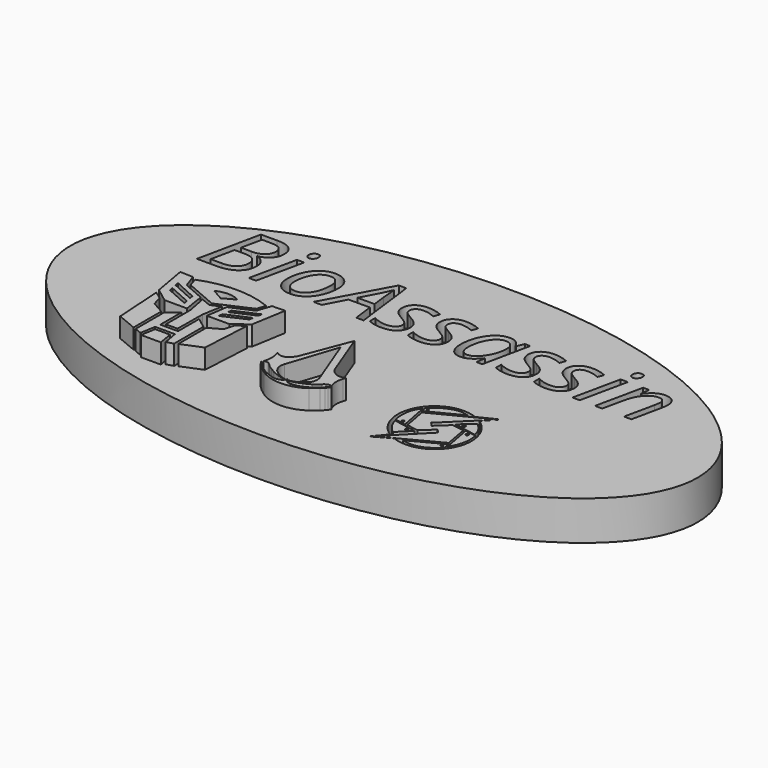
from build123d import *

# Parameters (mm, degrees)
F1_DEPTH     = 6.35
F3_DEPTH     = 3.175
F4_TEXT_SIZE = 14.3641968154
F5_DEPTH     = 3.175
F7_DEPTH     = 3.175
F8_R         = 0.1916506527
F8_R_2       = 0.1928443089
F8_R_3       = 0.2170281885
F8_R_4       = 0.2291424011
F8_R_5       = 0.2516270003
F8_R_6       = 0.1916500299
F9_DEPTH     = 3.175


# Not quite as in the source:
# - Text() gives the source's letters only with a copy of the font that has no kerning and outlines rounded to 1/6400 em; it was checked with that copy


with BuildPart() as f1:
    # F0 (on Top) → F1 (new body)
    with BuildSketch(Plane.XY):
        with BuildLine():
            add(Edge.make_bspline(
                [(-2.0761744499, 26.4380853623), (-2.0761744499, 70.4321758746), (-78.2761744499, 48.4351306184), (-154.4761744499, 26.4380853623), (-78.2761744499, 4.4410401062), (-2.0761744499, -17.5560051499), (-2.0761744499, 26.4380853623)],
                knots=[0, 0, 0, 2.0943951024, 2.0943951024, 4.1887902048, 4.1887902048, 6.2831853072, 6.2831853072, 6.2831853072], degree=2, weights=[1, 0.5, 1, 0.5, 1, 0.5, 1]))
        make_face()
    extrude(amount=F1_DEPTH)

    # F2 (on face) → F3 (join)
    with BuildSketch(Plane.XY.offset(6.35)):
        Polygon((-82.4147164822, 24.7203502804), (-84.5443084836, 24.7908383608), (-83.562836051, 19.2485265434), (-81.2740772963, 17.5208002329), (-77.6344388723, 17.5208002329), (-78.1894996762, 20.9758300334), (-81.6669389606, 22.4755033851), align=None)
        Polygon((-82.5627523526, 20.7187378721), (-78.9317861199, 19.0999638289), (-78.8153856993, 18.4600390494), (-82.4462398887, 20.0781971216), align=None, mode=Mode.SUBTRACT)
        Polygon((-82.7492848039, 21.5894449502), (-82.8499123454, 22.226523608), (-79.2003050447, 20.5615349114), (-79.0968462825, 19.9539288878), align=None, mode=Mode.SUBTRACT)
        with BuildLine():
            Line((-81.2787341385, 22.8053983301), (-76.0416015983, 20.5468432649))
            Line((-76.0416015983, 20.5468432649), (-70.7222604523, 22.9139946496))
            Line((-70.7222604523, 22.9139946496), (-70.2862739563, 24.3399571627))
            ThreePointArc((-70.2862739563, 24.3399571627), (-76.031431719, 25.4278744594), (-81.766679883, 24.2888703942))
            Line((-81.766679883, 24.2888703942), (-81.2787341385, 22.8053983301))
        make_face()
        with BuildLine():
            Line((-74.1477385163, 23.4021712095), (-76.0516747832, 22.3448332399))
            Line((-76.0516747832, 22.3448332399), (-77.9415145516, 23.4303679317))
            ThreePointArc((-77.9415145516, 23.4303679317), (-76.0411760601, 23.8805194576), (-74.1477385163, 23.4021712095))
        make_face(mode=Mode.SUBTRACT)
        Polygon((-68.4861242771, 19.2485265434), (-67.5502344966, 24.7908383608), (-69.6382522583, 24.7203502804), (-70.4108700156, 22.5014146417), (-73.9257629703, 20.937257823), (-74.4184702635, 17.5208002329), (-70.7782804966, 17.5208002329), align=None)
        Polygon((-73.2523426414, 18.4075301513), (-73.124319315, 19.0999638289), (-69.484680891, 20.7005254924), (-69.5944130421, 20.0781971216), align=None, mode=Mode.SUBTRACT)
        Polygon((-72.9846805334, 19.970158115), (-72.8859528899, 20.545469597), (-69.2050084472, 22.1835207194), (-69.3319365382, 21.605508402), align=None, mode=Mode.SUBTRACT)
        Polygon((-77.0146325231, 12.4494610354), (-75.1125067472, 12.4494610354), (-75.068205595, 17.4013171345), (-74.5082125068, 20.6776876003), (-76.0416015983, 20.0145617127), (-77.6344388723, 20.6776876003), (-77.0146325231, 17.4209345132), align=None)
        Polygon((-69.1682100296, 10.5674592778), (-68.7141045928, 18.5484457761), (-69.9991939274, 17.5798020878), (-70.4403966665, 15.9944351763), (-72.4175944924, 14.8910367861), (-72.4175944924, 9.2318430543), align=None)
        Polygon((-79.2059600353, 9.0901833028), (-78.0537128448, 8.614834398), (-77.6344388723, 11.0687091266), (-74.4305490002, 11.0687091266), (-73.9895477891, 8.6442539468), (-72.8844925761, 8.9761884883), (-72.8844925761, 14.8910367861), (-74.6236592531, 16.2018369883), (-74.6236592531, 11.9371591136), (-77.4938840032, 11.9371591136), (-77.4938840032, 16.1815242237), (-79.2059600353, 14.8910367861), align=None)
        Polygon((-82.1009427309, 17.5828840584), (-83.3817571402, 18.483851105), (-82.8867703676, 10.5674592778), (-79.6579048038, 9.2318430543), (-79.6579048038, 14.8325646296), (-81.674002111, 15.9943383187), align=None)
        Polygon((-77.6344388723, 8.2036182284), (-74.4305490002, 8.2036182284), (-74.8137384653, 10.5674592778), (-77.2304141556, 10.5674592778), align=None)
    extrude(amount=F3_DEPTH)

    # F4 (on face) → F5 (cut)
    with BuildSketch(Plane.XY.offset(6.35)):
        with Locations((-89.5551151694, 33.6692477039)):
            Text('BioAssassin', F4_TEXT_SIZE, font='Open Sans', font_style=FontStyle.ITALIC, text_align=(TextAlign.LEFT, TextAlign.BOTTOM))
    extrude(amount=-F5_DEPTH, mode=Mode.SUBTRACT)

    # F6 (on face) → F7 (join)
    with BuildSketch(Plane.XY.offset(6.35)):
        with BuildLine():
            Line((-52.6945255697, 16.3291338831), (-55.5437318981, 23.7856209278))
            Line((-55.5437318981, 23.7856209278), (-58.414824307, 16.3291338831))
            ThreePointArc((-58.414824307, 16.3291338831), (-58.8506670699, 15.5641376779), (-59.493497014, 14.9625167251))
            ThreePointArc((-59.493497014, 14.9625167251), (-60.1241290569, 14.8377622573), (-60.7547610998, 14.9625167251))
            Line((-60.7547610998, 14.9625167251), (-61.1454695463, 15.1783749461))
            Line((-61.1454695463, 15.1783749461), (-61.0354021192, 14.8442285135))
            ThreePointArc((-61.0354021192, 14.8442285135), (-60.8451342355, 13.5664848197), (-61.092838645, 12.2986230999))
            ThreePointArc((-61.092838645, 12.2986230999), (-60.6760960072, 12.4114563583), (-60.2593533695, 12.2986230999))
            ThreePointArc((-60.2593533695, 12.2986230999), (-60.0322026683, 12.1243368544), (-59.8218515515, 11.9301062077))
            ThreePointArc((-59.8218515515, 11.9301062077), (-59.4426166469, 11.5804195892), (-59.009861201, 11.2996660173))
            ThreePointArc((-59.009861201, 11.2996660173), (-58.5642308897, 11.0422791652), (-58.1313483417, 10.7639860362))
            Line((-58.1313483417, 10.7639860362), (-57.2099797428, 10.3997243568))
            Line((-57.2099797428, 10.3997243568), (-56.1814717948, 10.0997434929))
            Line((-56.1814717948, 10.0997434929), (-55.9638403356, 10.1530635729))
            ThreePointArc((-55.9638403356, 10.1530635729), (-56.972408552, 10.5343120692), (-57.8737519681, 11.1260386184))
            ThreePointArc((-57.8737519681, 11.1260386184), (-58.5074146767, 12.117024421), (-58.4797412157, 13.292956166))
            Line((-58.4797412157, 13.292956166), (-55.8136813343, 21.3448889554))
            Line((-55.8136813343, 21.3448889554), (-52.7151487768, 13.292956166))
            ThreePointArc((-52.7151487768, 13.292956166), (-52.573703275, 12.5315515324), (-52.7151487768, 11.7701468989))
            ThreePointArc((-52.7151487768, 11.7701468989), (-53.8074252425, 10.7152896987), (-55.220130831, 10.1584643126))
            Line((-55.220130831, 10.1584643126), (-55.220130831, 10.0887585431))
            Line((-55.220130831, 10.0887585431), (-55.0755619163, 10.0872691162))
            Line((-55.0755619163, 10.0872691162), (-54.926853627, 10.1157864556))
            ThreePointArc((-54.926853627, 10.1157864556), (-54.1330560104, 10.32589303), (-53.3758886158, 10.6436302885))
            ThreePointArc((-53.3758886158, 10.6436302885), (-52.8066194383, 10.8842523092), (-52.2688739002, 11.1888768151))
            ThreePointArc((-52.2688739002, 11.1888768151), (-51.8127052896, 11.5361639491), (-51.3793900609, 11.9115784764))
            ThreePointArc((-51.3793900609, 11.9115784764), (-51.1378053717, 12.1359126534), (-50.864636898, 12.32048776))
            ThreePointArc((-50.864636898, 12.32048776), (-50.4785850644, 12.4258280659), (-50.0925332308, 12.32048776))
            ThreePointArc((-50.0925332308, 12.32048776), (-50.3577581264, 13.5407270824), (-50.1651577652, 14.7745152935))
            Line((-50.1651577652, 14.7745152935), (-50.012268126, 15.2076985687))
            ThreePointArc((-50.012268126, 15.2076985687), (-50.9923047667, 15.017606853), (-51.923379302, 15.3777552769))
            ThreePointArc((-51.923379302, 15.3777552769), (-52.3847807438, 15.7919814398), (-52.6945255697, 16.3291338831))
        make_face()
        with BuildLine():
            Line((-60.4039542377, 11.1920423806), (-61.3175854087, 12.1777709574))
            Line((-61.3175854087, 12.1777709574), (-60.884796083, 11.471843347))
            Line((-60.884796083, 11.471843347), (-60.0586645305, 10.6787569821))
            Line((-60.0586645305, 10.6787569821), (-59.184871614, 10.0024132989))
            ThreePointArc((-59.184871614, 10.0024132989), (-55.5615715351, 8.9245454583), (-51.9603267312, 10.0739533082))
            Line((-51.9603267312, 10.0739533082), (-50.8481524885, 10.9758134931))
            Line((-50.8481524885, 10.9758134931), (-50.4277087748, 11.4089967683))
            Line((-50.4277087748, 11.4089967683), (-50.1728951931, 11.7020327598))
            Line((-50.1728951931, 11.7020327598), (-49.9053411186, 12.1479565278))
            Line((-49.9053411186, 12.1479565278), (-51.3832606375, 10.7592223212))
            Line((-51.3832606375, 10.7592223212), (-51.9632063806, 10.3787044063))
            Line((-51.9632063806, 10.3787044063), (-52.5084510446, 10.0647751242))
            Line((-52.5084510446, 10.0647751242), (-53.0867427588, 9.8169352859))
            Line((-53.0867427588, 9.8169352859), (-53.5989440978, 9.6682319418))
            Line((-53.5989440978, 9.6682319418), (-54.3010719121, 9.5893479884))
            ThreePointArc((-54.3010719121, 9.5893479884), (-54.8227626811, 9.5912851885), (-55.2867203951, 9.8298396915))
            ThreePointArc((-55.2867203951, 9.8298396915), (-55.5361325834, 10.0477630637), (-55.629555136, 10.3655196726))
            ThreePointArc((-55.629555136, 10.3655196726), (-55.7975668063, 9.9752291328), (-56.1223812401, 9.701276198))
            ThreePointArc((-56.1223812401, 9.701276198), (-56.7894545037, 9.5063378454), (-57.4794523418, 9.5893479884))
            Line((-57.4794523418, 9.5893479884), (-57.8759945929, 9.7215287387))
            Line((-57.8759945929, 9.7215287387), (-58.3386272192, 9.8867546767))
            Line((-58.3386272192, 9.8867546767), (-58.9169189334, 10.1180719212))
            Line((-58.9169189334, 10.1180719212), (-59.3465082347, 10.3989560157))
            Line((-59.3465082347, 10.3989560157), (-59.7265288234, 10.6633184478))
            Line((-59.7265288234, 10.6633184478), (-60.4039542377, 11.1920423806))
        make_face()
    extrude(amount=F7_DEPTH)

    # F8 (on face) → F9 (cut)
    with BuildSketch(Plane.XY.offset(6.35)):
        with BuildLine():
            Line((-37.2062667566, 16.5136284461), (-35.2589562535, 18.3137860149))
            Line((-35.2589562535, 18.3137860149), (-33.299356699, 18.0459283292))
            Line((-33.299356699, 18.0459283292), (-32.6120853424, 14.189902693))
            Line((-32.6120853424, 14.189902693), (-38.8427486068, 10.9035546382))
            ThreePointArc((-38.8427486068, 10.9035546382), (-38.801494898, 10.886636332), (-38.7601148824, 10.8700293489))
            ThreePointArc((-38.7601148824, 10.8700293489), (-31.3246717169, 13.6439376984), (-33.3356498177, 21.3209390451))
            ThreePointArc((-33.3356498177, 21.3209390451), (-33.3859478171, 21.3535047148), (-33.4365729908, 21.3855594083))
            Line((-33.4365729908, 21.3855594083), (-37.7934388816, 17.1122867614))
            Line((-37.7934388816, 17.1122867614), (-37.2062667566, 16.5136284461))
        make_face()
        with BuildLine():
            Line((-37.594482869, 11.1393940492), (-32.3966816068, 13.8809615746))
            Line((-32.3966816068, 13.8809615746), (-32.2297140956, 12.9604581743))
            ThreePointArc((-32.2297140956, 12.9604581743), (-32.8177926393, 12.2755847137), (-33.5424952209, 11.7373522371))
            ThreePointArc((-33.5424952209, 11.7373522371), (-35.4998134999, 10.973002042), (-37.594482869, 11.1393940492))
        make_face(mode=Mode.SUBTRACT)
        with BuildLine():
            Line((-32.092358917, 13.3310221136), (-32.9998425444, 18.1519521318))
            Line((-32.9998425444, 18.1519521318), (-31.1933811754, 17.8243145347))
            ThreePointArc((-31.1933811754, 17.8243145347), (-31.1749344716, 15.4840479614), (-32.092358917, 13.3310221136))
        make_face(mode=Mode.SUBTRACT)
        with BuildLine():
            ThreePointArc((-33.0749601126, 20.530147478), (-32.0100919257, 19.4404554098), (-31.4502753317, 18.0234238505))
            Line((-31.4502753317, 18.0234238505), (-35.1080857217, 18.6868403107))
            Line((-35.1080857217, 18.6868403107), (-33.0749601126, 20.530147478))
        make_face(mode=Mode.SUBTRACT)
        with BuildLine():
            ThreePointArc((-39.8774278669, 11.3796028695), (-39.7679254917, 11.3090182611), (-39.6568980394, 11.2408577011))
            Line((-39.6568980394, 11.2408577011), (-38.6616959256, 12.2690652771))
            Line((-38.6616959256, 12.2690652771), (-35.3911779821, 15.5759230256))
            Line((-35.3911779821, 15.5759230256), (-35.9925856615, 16.1707217005))
            Line((-35.9925856615, 16.1707217005), (-37.8816947341, 14.4261745736))
            Line((-37.8816947341, 14.4261745736), (-39.7465229034, 14.7735448554))
            Line((-39.7465229034, 14.7735448554), (-40.4524542391, 18.5989812016))
            Line((-40.4524542391, 18.5989812016), (-34.2745172378, 21.7714778578))
            ThreePointArc((-34.2745172378, 21.7714778578), (-34.358147481, 21.806615463), (-34.4423057308, 21.8404689392))
            ThreePointArc((-34.4423057308, 21.8404689392), (-41.8709851997, 19.0577781597), (-39.8774278669, 11.3796028695))
        make_face()
        with BuildLine():
            Line((-41.0268865526, 19.4920543581), (-40.0944799185, 14.7036602721))
            Line((-40.0944799185, 14.7036602721), (-41.8187193573, 14.9960657582))
            ThreePointArc((-41.8187193573, 14.9960657582), (-42.0239693866, 16.0254156367), (-41.9873781502, 17.0743912458))
            ThreePointArc((-41.9873781502, 17.0743912458), (-41.725389085, 18.3699320534), (-41.0268865526, 19.4920543581))
        make_face(mode=Mode.SUBTRACT)
        with BuildLine():
            Line((-41.7237691581, 14.7465411574), (-38.0216958323, 14.0534586363))
            Line((-38.0216958323, 14.0534586363), (-39.9888940156, 12.1194440871))
            ThreePointArc((-39.9888940156, 12.1194440871), (-41.0746850488, 13.2887969632), (-41.7237691581, 14.7465411574))
        make_face(mode=Mode.SUBTRACT)
        with BuildLine():
            Line((-35.4709093757, 21.5859033874), (-40.6893827021, 18.9061108977))
            Line((-40.6893827021, 18.9061108977), (-40.8539904644, 19.7514575592))
            ThreePointArc((-40.8539904644, 19.7514575592), (-39.3739670495, 21.0063853763), (-37.578843534, 21.7431653291))
            ThreePointArc((-37.578843534, 21.7431653291), (-36.5144033578, 21.8049154237), (-35.4709093757, 21.5859033874))
        make_face(mode=Mode.SUBTRACT)
        with Locations((-40.3108000755, 19.5802841336)):
            Circle(F8_R)
        with Locations((-40.8544950187, 15.2746196836)):
            Circle(F8_R_2)
        with Locations((-39.0651710331, 13.7769915164)):
            Circle(F8_R_3)
        with Locations((-32.2268418968, 17.4432266504)):
            Circle(F8_R_4)
        with Locations((-33.9774601161, 19.0271213651)):
            Circle(F8_R_5)
        with Locations((-32.8161455691, 13.0735943094)):
            Circle(F8_R_6)
        with BuildLine():
            Line((-31.6898748279, 23.098744452), (-33.4365729908, 21.3855594083))
            ThreePointArc((-33.4365729908, 21.3855594083), (-33.3859478171, 21.3535047148), (-33.3356498177, 21.3209390451))
            Line((-33.3356498177, 21.3209390451), (-31.4274765551, 23.3315490186))
            Line((-31.4274765551, 23.3315490186), (-34.4423057308, 21.8404689392))
            ThreePointArc((-34.4423057308, 21.8404689392), (-34.358147481, 21.806615463), (-34.2745172378, 21.7714778578))
            Line((-34.2745172378, 21.7714778578), (-31.6898748279, 23.098744452))
        make_face()
        with BuildLine():
            ThreePointArc((-38.7601148824, 10.8700293489), (-38.801494898, 10.886636332), (-38.8427486068, 10.9035546382))
            Line((-38.8427486068, 10.9035546382), (-41.1730110645, 9.6744634211))
            Line((-41.1730110645, 9.6744634211), (-39.6568980394, 11.2408577011))
            ThreePointArc((-39.6568980394, 11.2408577011), (-39.7679254917, 11.3090182611), (-39.8774278669, 11.3796028695))
            Line((-39.8774278669, 11.3796028695), (-41.5874384344, 9.2834802344))
            Line((-41.5874384344, 9.2834802344), (-38.7601148824, 10.8700293489))
        make_face()
    extrude(amount=-F9_DEPTH, mode=Mode.SUBTRACT)


solid = f1.part
